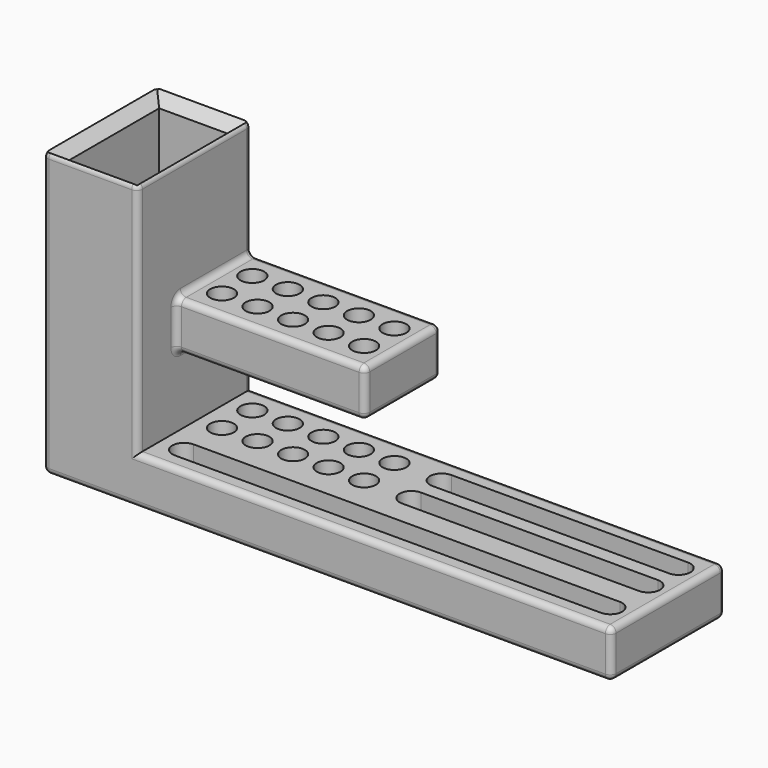
from build123d import *

# Parameters (mm, degrees)
F1_DEPTH      = 76.2
F0_W          = 101.6
F0_H          = 25.4
F2_DEPTH      = 50.8
F3_T          = -6.604
F4_R          = 3.175
F5_R          = 6.35
F6_DEPTH      = 95.25
F7_W          = 119.4815961644
F7_H          = 43.3120825328
F8_DEPTH      = 6.35
F10_DEPTH     = 19.05
F11_DEPTH     = 25.4
F12_DEPTH     = 25.4
F13_T1_DEPTH  = 62.992
F13_T3_DEPTH  = 37.592
F13_T9_DEPTH  = 79.3221869736
F13_T13_DEPTH = 53.9221869736
F13_T20_DEPTH = 79.3221869736
F13_T24_DEPTH = 53.9221869736
F13_T31_DEPTH = 53.9221869736
F13_T35_DEPTH = 79.3221869736
F13_T42_DEPTH = 79.3221869736
F13_T46_DEPTH = 53.9221869736


# Not quite as in the source:
# - a fillet or chamfer that OpenCascade refuses, or shapes differently, is made with other operations: its cross-section is extruded or revolved along the edge and cut away or added


with BuildPart() as f1:
    # F0 (on Front) → F1 (new body)
    with BuildSketch(Plane.XZ):
        Polygon((-152.4, 25.4), (-152.4, 0), (152.4, 0), (152.4, 25.4), (-101.6, 25.4), align=None)
        Polygon((-152.4, 152.4), (-152.4, 25.4), (-101.6, 25.4), (-101.6, 63.5), (-101.6, 88.9), (-101.6, 152.4), align=None)
    extrude(amount=F1_DEPTH)

    # F0 (on Front) → F2 (join)
    with BuildSketch(Plane.XZ):
        with Locations((-50.8, 76.2)):
            Rectangle(F0_W, F0_H)
    extrude(amount=F2_DEPTH)

    # F3
    f3_openings = [f1.faces().sort_by_distance(p)[0] for p in [
        (-127, -38.1, 152.4),
    ]]
    offset(amount=F3_T, openings=f3_openings, kind=Kind.INTERSECTION)

    # F4
    f4_edges = [f1.edges().sort_by_distance(p)[0] for p in [
        (-152.4, -76.2, 76.2),
        (-101.6, -76.2, 88.9),
        (0, -50.8, 76.2),
        (0, 0, 76.2),
        (-152.4, 0, 76.2),
        (-101.6, 0, 44.45),
        (-101.6, 0, 120.65),
        (152.4, 0, 12.7),
        (152.4, -76.2, 12.7),
        (-101.6, -50.8, 76.2),
        (-50.8, 0, 88.9),
        (-50.8, -50.8, 88.9),
        (-50.8, -50.8, 63.5),
        (-50.8, 0, 63.5),
        (25.4, 0, 25.4),
        (0, -76.2, 0),
        (25.4, -76.2, 25.4),
        (152.4, -38.1, 25.4),
        (152.4, -38.1, 0),
        (0, 0, 0),
        (-152.4, -38.1, 0),
        (0, -25.4, 63.5),
        (0, -25.4, 88.9),
        (-101.6, -38.1, 152.4),
        (-152.4, -38.1, 152.4),
        (-127, -76.2, 152.4),
        (-127, 0, 152.4),
        (-101.6, -25.4, 63.5),
        (-101.6, -25.4, 88.9),
    ]]
    fillet(f4_edges, radius=F4_R)

    # F5 (on Top) → F6 (cut)
    with BuildSketch(Plane.XY):
        with Locations((-12.7, -35.56)):
            Circle(F5_R)
        with Locations((-12.7, -15.24)):
            Circle(F5_R)
        with Locations((-31.75, -35.56)):
            Circle(F5_R)
        with Locations((-31.75, -15.24)):
            Circle(F5_R)
        with Locations((-50.8, -35.56)):
            Circle(F5_R)
        with Locations((-50.8, -15.24)):
            Circle(F5_R)
        with Locations((-69.85, -35.56)):
            Circle(F5_R)
        with Locations((-69.85, -15.24)):
            Circle(F5_R)
        with Locations((-88.9, -35.56)):
            Circle(F5_R)
        with Locations((-88.9, -15.24)):
            Circle(F5_R)
    extrude(amount=F6_DEPTH, mode=Mode.SUBTRACT)

    # F7 (on face) → F8 (join)
    with BuildSketch(Plane(origin=(0, 0, 0), x_dir=(1, 0, 0), z_dir=(0, 0, -1))):
        with Locations((-48.7527609803, 27.0967211109)):
            Rectangle(F7_W, F7_H)
    extrude(amount=-F8_DEPTH)

    # F9 (on face) → F10 (cut)
    with BuildSketch(Plane.XY.offset(25.4)):
        with BuildLine():
            ThreePointArc((-88.9, -54.61), (-84.4098719395, -56.4698719395), (-82.55, -60.96))
            ThreePointArc((-82.55, -60.96), (-84.4098719395, -65.4501280605), (-88.9, -67.31))
            Line((-88.9, -67.31), (139.7, -67.31))
            ThreePointArc((139.7, -67.31), (133.35, -60.96), (139.7, -54.61))
            Line((139.7, -54.61), (-88.9, -54.61))
        make_face()
        with BuildLine():
            ThreePointArc((12.7, -29.21), (17.1901280605, -31.0698719395), (19.05, -35.56))
            ThreePointArc((19.05, -35.56), (17.1901280605, -40.0501280605), (12.7, -41.91))
            Line((12.7, -41.91), (139.7, -41.91))
            ThreePointArc((139.7, -41.91), (133.35, -35.56), (139.7, -29.21))
            Line((139.7, -29.21), (12.7, -29.21))
        make_face()
        with BuildLine():
            ThreePointArc((12.7, -8.89), (17.1901280605, -10.7498719395), (19.05, -15.24))
            ThreePointArc((19.05, -15.24), (17.1901280605, -19.7301280605), (12.7, -21.59))
            Line((12.7, -21.59), (139.7, -21.59))
            ThreePointArc((139.7, -21.59), (133.35, -15.24), (139.7, -8.89))
            Line((139.7, -8.89), (12.7, -8.89))
        make_face()
        with BuildLine():
            ThreePointArc((146.05, -60.96), (144.1901280605, -56.4698719395), (139.7, -54.61))
            ThreePointArc((139.7, -54.61), (133.35, -60.96), (139.7, -67.31))
            ThreePointArc((139.7, -67.31), (144.1901280605, -65.4501280605), (146.05, -60.96))
        make_face()
        with BuildLine():
            ThreePointArc((146.05, -15.24), (144.1901280605, -10.7498719395), (139.7, -8.89))
            ThreePointArc((139.7, -8.89), (133.35, -15.24), (139.7, -21.59))
            ThreePointArc((139.7, -21.59), (144.1901280605, -19.7301280605), (146.05, -15.24))
        make_face()
        with BuildLine():
            ThreePointArc((146.05, -35.56), (144.1901280605, -31.0698719395), (139.7, -29.21))
            ThreePointArc((139.7, -29.21), (133.35, -35.56), (139.7, -41.91))
            ThreePointArc((139.7, -41.91), (144.1901280605, -40.0501280605), (146.05, -35.56))
        make_face()
        with BuildLine():
            ThreePointArc((12.7, -41.91), (17.1901280605, -40.0501280605), (19.05, -35.56))
            ThreePointArc((19.05, -35.56), (17.1901280605, -31.0698719395), (12.7, -29.21))
            ThreePointArc((12.7, -29.21), (6.35, -35.56), (12.7, -41.91))
        make_face()
        with BuildLine():
            ThreePointArc((12.7, -21.59), (17.1901280605, -19.7301280605), (19.05, -15.24))
            ThreePointArc((19.05, -15.24), (17.1901280605, -10.7498719395), (12.7, -8.89))
            ThreePointArc((12.7, -8.89), (6.35, -15.24), (12.7, -21.59))
        make_face()
        with BuildLine():
            ThreePointArc((-88.9, -67.31), (-84.4098719395, -65.4501280605), (-82.55, -60.96))
            ThreePointArc((-82.55, -60.96), (-84.4098719395, -56.4698719395), (-88.9, -54.61))
            ThreePointArc((-88.9, -54.61), (-95.25, -60.96), (-88.9, -67.31))
        make_face()
    extrude(amount=-F10_DEPTH, mode=Mode.SUBTRACT)

    # F11 (add): a face of the model
    f11_faces = [f1.faces().sort_by_distance(p)[0] for p in [
        (-50.8, -25.4, 88.9),
    ]]
    extrude(f11_faces, amount=-F11_DEPTH)

    # F12 (add): a face of the model
    f12_faces = [f1.faces().sort_by_distance(p)[0] for p in [
        (-98.9963064096, -38.1, 25.4),
    ]]
    extrude(f12_faces, amount=-F12_DEPTH)

    # F13: chamfer of 6.35 on 20 edges, made by hand

    # F13_s2 → F13_t1 (cut)
    with BuildSketch(Plane.XZ.offset(6.604)):
        with BuildLine():
            Line((-101.6743948776, 152.5796051224), (-108.3836051224, 145.8703948776))
            Line((-108.3836051224, 145.8703948776), (-108.5106051224, 145.8703948776))
            ThreePointArc((-108.5106051224, 145.8703948776), (-108.331, 149.1351974388), (-108.331, 152.4))
            Line((-108.331, 152.4), (-108.204, 152.527))
            ThreePointArc((-108.204, 152.527), (-104.9391974388, 152.527), (-101.6743948776, 152.7066051224))
            Line((-101.6743948776, 152.7066051224), (-101.6743948776, 152.5796051224))
        make_face()
        with BuildLine():
            Line((-152.3256051224, 152.5796051224), (-145.6163948776, 145.8703948776))
            Line((-145.6163948776, 145.8703948776), (-145.4893948776, 145.8703948776))
            ThreePointArc((-145.4893948776, 145.8703948776), (-145.669, 149.1351974388), (-145.669, 152.4))
            Line((-145.669, 152.4), (-145.796, 152.527))
            ThreePointArc((-145.796, 152.527), (-149.0608025612, 152.527), (-152.3256051224, 152.7066051224))
            Line((-152.3256051224, 152.7066051224), (-152.3256051224, 152.5796051224))
        make_face()
    extrude(amount=F13_T1_DEPTH, mode=Mode.SUBTRACT)

    # F13_s4 → F13_t3 (cut)
    with BuildSketch(Plane.YZ.offset(-145.796)):
        with BuildLine():
            Line((-0.0743948776, 152.5796051224), (-6.7836051224, 145.8703948776))
            Line((-6.7836051224, 145.8703948776), (-6.9106051224, 145.8703948776))
            ThreePointArc((-6.9106051224, 145.8703948776), (-6.731, 149.1351974388), (-6.731, 152.4))
            Line((-6.731, 152.4), (-6.604, 152.527))
            ThreePointArc((-6.604, 152.527), (-3.3391974388, 152.527), (-0.0743948776, 152.7066051224))
            Line((-0.0743948776, 152.7066051224), (-0.0743948776, 152.5796051224))
        make_face()
        with BuildLine():
            Line((-76.1256051224, 152.5796051224), (-69.4163948776, 145.8703948776))
            Line((-69.4163948776, 145.8703948776), (-69.2893948776, 145.8703948776))
            ThreePointArc((-69.2893948776, 145.8703948776), (-69.469, 149.1351974388), (-69.469, 152.4))
            Line((-69.469, 152.4), (-69.596, 152.527))
            ThreePointArc((-69.596, 152.527), (-72.8608025612, 152.527), (-76.1256051224, 152.7066051224))
            Line((-76.1256051224, 152.7066051224), (-76.1256051224, 152.5796051224))
        make_face()
    extrude(amount=F13_T3_DEPTH, mode=Mode.SUBTRACT)


with BuildPart() as f13_tool7:
    # F13_s8 → F13_t9 (new body)
    with BuildSketch(Plane.XZ.offset(85.9261869736)):
        with BuildLine():
            Line((-101.6743948776, 152.5796051224), (-108.3836051224, 145.8703948776))
            Line((-108.3836051224, 145.8703948776), (-108.5106051224, 145.8703948776))
            ThreePointArc((-108.5106051224, 145.8703948776), (-108.331, 149.1351974388), (-108.331, 152.4))
            Line((-108.331, 152.4), (-108.204, 152.527))
            ThreePointArc((-108.204, 152.527), (-104.9391974388, 152.527), (-101.6743948776, 152.7066051224))
            Line((-101.6743948776, 152.7066051224), (-101.6743948776, 152.5796051224))
        make_face()
    extrude(amount=-F13_T9_DEPTH)

    split(bisect_by=Plane.XZ.offset(69.596), keep=Keep.TOP)


with BuildPart() as f13_tool11:
    # F13_s12 → F13_t13 (new body)
    with BuildSketch(Plane.YZ.offset(-91.8738130264)):
        with BuildLine():
            Line((-76.1256051224, 152.5796051224), (-69.4163948776, 145.8703948776))
            Line((-69.4163948776, 145.8703948776), (-69.2893948776, 145.8703948776))
            ThreePointArc((-69.2893948776, 145.8703948776), (-69.469, 149.1351974388), (-69.469, 152.4))
            Line((-69.469, 152.4), (-69.596, 152.527))
            ThreePointArc((-69.596, 152.527), (-72.8608025612, 152.527), (-76.1256051224, 152.7066051224))
            Line((-76.1256051224, 152.7066051224), (-76.1256051224, 152.5796051224))
        make_face()
    extrude(amount=-F13_T13_DEPTH)

    split(bisect_by=Plane.YZ.offset(-108.204), keep=Keep.TOP)


with BuildPart() as f13_tool7_1:
    add(f13_tool7.part)

    # F13_t15: intersect F13_tool11
    add(f13_tool11.part, mode=Mode.INTERSECT)


with BuildPart() as f1_1:
    add(f1.part)

    # F13_t5: cut F13_tool7
    add(f13_tool7_1.part, mode=Mode.SUBTRACT)


with BuildPart() as f13_tool18:
    # F13_s19 → F13_t20 (new body)
    with BuildSketch(Plane.XZ.offset(69.596)):
        with BuildLine():
            Line((-101.6743948776, 152.5796051224), (-108.3836051224, 145.8703948776))
            Line((-108.3836051224, 145.8703948776), (-108.5106051224, 145.8703948776))
            ThreePointArc((-108.5106051224, 145.8703948776), (-108.331, 149.1351974388), (-108.331, 152.4))
            Line((-108.331, 152.4), (-108.204, 152.527))
            ThreePointArc((-108.204, 152.527), (-104.9391974388, 152.527), (-101.6743948776, 152.7066051224))
            Line((-101.6743948776, 152.7066051224), (-101.6743948776, 152.5796051224))
        make_face()
    extrude(amount=-F13_T20_DEPTH)

    split(bisect_by=Plane.XZ.offset(6.604), keep=Keep.BOTTOM)


with BuildPart() as f13_tool22:
    # F13_s23 → F13_t24 (new body)
    with BuildSketch(Plane.YZ.offset(-91.8738130264)):
        with BuildLine():
            Line((-0.0743948776, 152.5796051224), (-6.7836051224, 145.8703948776))
            Line((-6.7836051224, 145.8703948776), (-6.9106051224, 145.8703948776))
            ThreePointArc((-6.9106051224, 145.8703948776), (-6.731, 149.1351974388), (-6.731, 152.4))
            Line((-6.731, 152.4), (-6.604, 152.527))
            ThreePointArc((-6.604, 152.527), (-3.3391974388, 152.527), (-0.0743948776, 152.7066051224))
            Line((-0.0743948776, 152.7066051224), (-0.0743948776, 152.5796051224))
        make_face()
    extrude(amount=-F13_T24_DEPTH)

    split(bisect_by=Plane.YZ.offset(-108.204), keep=Keep.TOP)


with BuildPart() as f13_tool18_1:
    add(f13_tool18.part)

    # F13_t26: intersect F13_tool22
    add(f13_tool22.part, mode=Mode.INTERSECT)


with BuildPart() as f1_2:
    add(f1_1.part)

    # F13_t16: cut F13_tool18
    add(f13_tool18_1.part, mode=Mode.SUBTRACT)


with BuildPart() as f13_tool29:
    # F13_s30 → F13_t31 (new body)
    with BuildSketch(Plane.YZ.offset(-108.204)):
        with BuildLine():
            Line((-0.0743948776, 152.5796051224), (-6.7836051224, 145.8703948776))
            Line((-6.7836051224, 145.8703948776), (-6.9106051224, 145.8703948776))
            ThreePointArc((-6.9106051224, 145.8703948776), (-6.731, 149.1351974388), (-6.731, 152.4))
            Line((-6.731, 152.4), (-6.604, 152.527))
            ThreePointArc((-6.604, 152.527), (-3.3391974388, 152.527), (-0.0743948776, 152.7066051224))
            Line((-0.0743948776, 152.7066051224), (-0.0743948776, 152.5796051224))
        make_face()
    extrude(amount=-F13_T31_DEPTH)

    split(bisect_by=Plane.YZ.offset(-145.796), keep=Keep.BOTTOM)


with BuildPart() as f13_tool33:
    # F13_s34 → F13_t35 (new body)
    with BuildSketch(Plane.XZ.offset(-9.7261869736)):
        with BuildLine():
            Line((-152.3256051224, 152.5796051224), (-145.6163948776, 145.8703948776))
            Line((-145.6163948776, 145.8703948776), (-145.4893948776, 145.8703948776))
            ThreePointArc((-145.4893948776, 145.8703948776), (-145.669, 149.1351974388), (-145.669, 152.4))
            Line((-145.669, 152.4), (-145.796, 152.527))
            ThreePointArc((-145.796, 152.527), (-149.0608025612, 152.527), (-152.3256051224, 152.7066051224))
            Line((-152.3256051224, 152.7066051224), (-152.3256051224, 152.5796051224))
        make_face()
    extrude(amount=F13_T35_DEPTH)

    split(bisect_by=Plane.XZ.offset(6.604), keep=Keep.BOTTOM)


with BuildPart() as f13_tool29_1:
    add(f13_tool29.part)

    # F13_t37: intersect F13_tool33
    add(f13_tool33.part, mode=Mode.INTERSECT)


with BuildPart() as f1_3:
    add(f1_2.part)

    # F13_t27: cut F13_tool29
    add(f13_tool29_1.part, mode=Mode.SUBTRACT)


with BuildPart() as f13_tool40:
    # F13_s41 → F13_t42 (new body)
    with BuildSketch(Plane.XZ.offset(6.604)):
        with BuildLine():
            Line((-152.3256051224, 152.5796051224), (-145.6163948776, 145.8703948776))
            Line((-145.6163948776, 145.8703948776), (-145.4893948776, 145.8703948776))
            ThreePointArc((-145.4893948776, 145.8703948776), (-145.669, 149.1351974388), (-145.669, 152.4))
            Line((-145.669, 152.4), (-145.796, 152.527))
            ThreePointArc((-145.796, 152.527), (-149.0608025612, 152.527), (-152.3256051224, 152.7066051224))
            Line((-152.3256051224, 152.7066051224), (-152.3256051224, 152.5796051224))
        make_face()
    extrude(amount=F13_T42_DEPTH)

    split(bisect_by=Plane.XZ.offset(69.596), keep=Keep.TOP)


with BuildPart() as f13_tool44:
    # F13_s45 → F13_t46 (new body)
    with BuildSketch(Plane.YZ.offset(-108.204)):
        with BuildLine():
            Line((-76.1256051224, 152.5796051224), (-69.4163948776, 145.8703948776))
            Line((-69.4163948776, 145.8703948776), (-69.2893948776, 145.8703948776))
            ThreePointArc((-69.2893948776, 145.8703948776), (-69.469, 149.1351974388), (-69.469, 152.4))
            Line((-69.469, 152.4), (-69.596, 152.527))
            ThreePointArc((-69.596, 152.527), (-72.8608025612, 152.527), (-76.1256051224, 152.7066051224))
            Line((-76.1256051224, 152.7066051224), (-76.1256051224, 152.5796051224))
        make_face()
    extrude(amount=-F13_T46_DEPTH)

    split(bisect_by=Plane.YZ.offset(-145.796), keep=Keep.BOTTOM)


with BuildPart() as f13_tool40_1:
    add(f13_tool40.part)

    # F13_t48: intersect F13_tool44
    add(f13_tool44.part, mode=Mode.INTERSECT)


with BuildPart() as f1_4:
    add(f1_3.part)

    # F13_t38: cut F13_tool40
    add(f13_tool40_1.part, mode=Mode.SUBTRACT)


solid = f1_4.part
